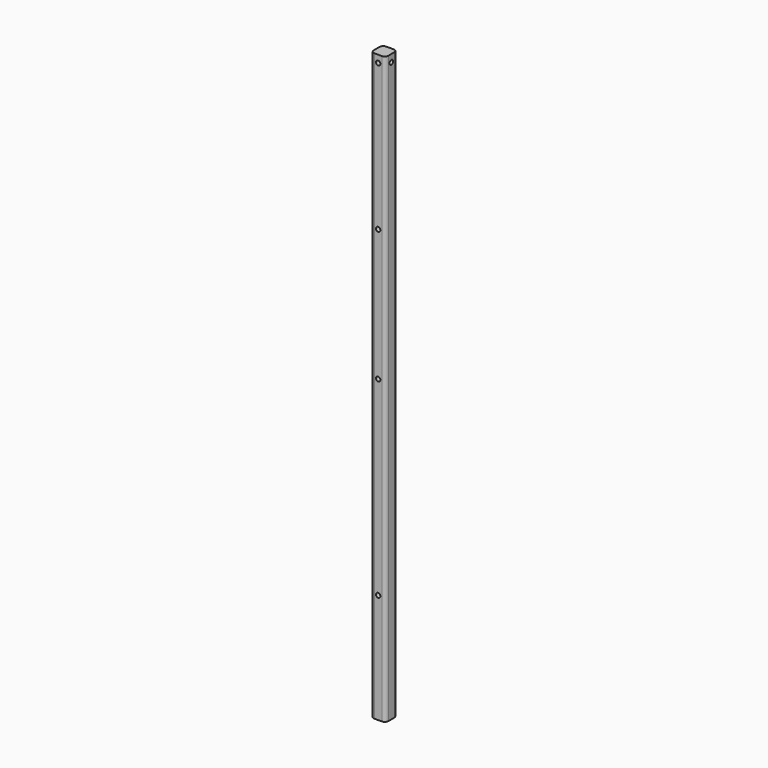
from build123d import *

# Parameters (mm, degrees)
F1_DEPTH = 1016
F3_DEPTH = 25.4
F5_DEPTH = 25.4
F2_R     = 3.81
F6_DEPTH = 25.4
F7_DEPTH = 25.4


# Not quite as in the source:
# - a feature names something its author has since deleted; it is built from what else it names


with BuildPart() as f1:
    # F0 (on Top) → F1 (new body)
    with BuildSketch(Plane.XY):
        with BuildLine():
            ThreePointArc((12.7, 6.35), (10.8401280605, 10.8401280605), (6.35, 12.7))
            Line((6.35, 12.7), (-6.35, 12.7))
            ThreePointArc((-6.35, 12.7), (-10.8401280605, 10.8401280605), (-12.7, 6.35))
            Line((-12.7, 6.35), (-12.7, -6.35))
            ThreePointArc((-12.7, -6.35), (-10.8401280605, -10.8401280605), (-6.35, -12.7))
            Line((-6.35, -12.7), (6.35, -12.7))
            ThreePointArc((6.35, -12.7), (10.8401280605, -10.8401280605), (12.7, -6.35))
            Line((12.7, -6.35), (12.7, 6.35))
        make_face()
    extrude(amount=F1_DEPTH)

    # F2 (on face) → F3 (cut)
    with BuildSketch(Plane.XZ.offset(12.7)):
        with BuildLine():
            ThreePointArc((3.81, 1003.3), (2.6940768363, 1005.9940768363), (0, 1007.11))
            ThreePointArc((0, 1007.11), (-2.6940768363, 1000.6059231637), (3.81, 1003.3))
        make_face()
    extrude(amount=-F3_DEPTH, mode=Mode.SUBTRACT)

    # F4 (on face) → F5 (cut)
    with BuildSketch(Plane.YZ.offset(12.7)):
        with BuildLine():
            ThreePointArc((3.81, 1003.3), (2.6940768363, 1005.9940768363), (0, 1007.11))
            ThreePointArc((0, 1007.11), (-2.6940768363, 1000.6059231637), (3.81, 1003.3))
        make_face()
    extrude(amount=-F5_DEPTH, mode=Mode.SUBTRACT)

    # F2 (on face) → F6 (cut)
    with BuildSketch(Plane.XZ.offset(12.7)):
        with Locations((0, 749.3)):
            Circle(F2_R)
        with Locations((0, 520.7)):
            Circle(F2_R)
    extrude(amount=-F6_DEPTH, mode=Mode.SUBTRACT)

    # F2 (on face) → F7 (cut)
    with BuildSketch(Plane.XZ.offset(12.7)):
        with Locations((0, 190.5)):
            Circle(F2_R)
    extrude(amount=-F7_DEPTH, mode=Mode.SUBTRACT)


solid = f1.part
